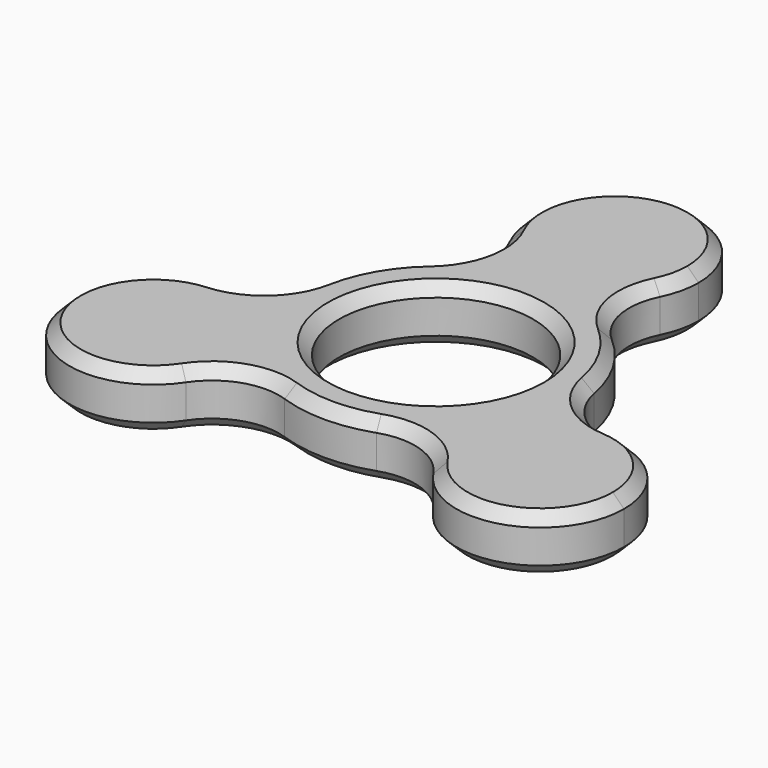
from build123d import *

# Parameters (mm, degrees)
F0_R     = 11.0363
F1_DEPTH = 6.35
F2_SIZE  = 1.27


# Not quite as in the source:
# - a feature names something its author has since deleted; it is built from what else it names


with BuildPart() as f1:
    # F0 (on Top) → F1 (new body)
    with BuildSketch(Plane.XY):
        with BuildLine():
            ThreePointArc((13.7481534459, -7.9374997215), (15.334072534, -4.1087521857), (15.875, 0))
            ThreePointArc((15.875, 0), (15.8042735617, 1.4968507561), (15.592724449, 2.9803639471))
            ThreePointArc((15.592724449, 2.9803639471), (13.7481532851, 7.9375), (10.3774331152, 12.0135135135))
            ThreePointArc((10.3774331152, 12.0135135135), (5.5362937901, 14.8783425176), (-1.09e-08, 15.875))
            ThreePointArc((-1.09e-08, 15.875), (-5.5362938003, 14.8783425138), (-10.3774331152, 12.0135135135))
            ThreePointArc((-10.3774331152, 12.0135135135), (-13.7481532851, 7.9375), (-15.592724449, 2.9803639471))
            ThreePointArc((-15.592724449, 2.9803639471), (-15.6531695071, -2.6446000421), (-13.7481534335, -7.9374997429))
            ThreePointArc((-13.7481534335, -7.9374997429), (-10.1168758016, -12.2337422327), (-5.2152913338, -14.9938774606))
            ThreePointArc((-5.2152913338, -14.9938774606), (0, -15.875), (5.2152913338, -14.9938774606))
            ThreePointArc((5.2152913338, -14.9938774606), (10.1168758111, -12.2337422248), (13.7481534459, -7.9374997215))
        make_face()
        Circle(F0_R, mode=Mode.SUBTRACT)
        with BuildLine():
            ThreePointArc((15.592724449, 2.9803639471), (15.8042735617, 1.4968507561), (15.875, 0))
            ThreePointArc((15.875, 0), (15.334072534, -4.1087521857), (13.7481534459, -7.9374997215))
            ThreePointArc((13.7481534459, -7.9374997215), (17.4968931029, -4.3051053849), (22.5971491052, -3.1939229768))
            ThreePointArc((22.5971491052, -3.1939229768), (18.038469294, -1.3052898819), (15.592724449, 2.9803639471))
        make_face()
        with BuildLine():
            ThreePointArc((14.0645929883, -17.9727436898), (12.4767771707, -13.0002009006), (13.7481534459, -7.9374997215))
            ThreePointArc((13.7481534459, -7.9374997215), (10.1168758111, -12.2337422248), (5.2152913338, -14.9938774606))
            ThreePointArc((5.2152913338, -14.9938774606), (10.149648844, -14.9691277131), (14.0645929883, -17.9727436898))
        make_face()
        with BuildLine():
            ThreePointArc((22.5971491052, -3.1939229768), (17.4968931029, -4.3051053849), (13.7481534459, -7.9374997215))
            ThreePointArc((13.7481534459, -7.9374997215), (12.4767771707, -13.0002009006), (14.0645929883, -17.9727436898))
            ThreePointArc((14.0645929883, -17.9727436898), (24.751043908, -21.81817506), (31.5220452561, -12.7))
            ThreePointArc((31.5220452561, -12.7), (28.9411655806, -6.1804280878), (22.5971491052, -3.1939229768))
        make_face()
        with BuildLine():
            ThreePointArc((-1.09e-08, 15.875), (5.5362937901, 14.8783425176), (10.3774331152, 12.0135135135))
            ThreePointArc((10.3774331152, 12.0135135135), (7.88882045, 16.274417595), (8.5325561169, 21.1666666667))
            ThreePointArc((8.5325561169, 21.1666666667), (5.0201157809, 17.3053065193), (-1.09e-08, 15.875))
        make_face()
        with BuildLine():
            ThreePointArc((-10.3774331152, 12.0135135135), (-5.5362938003, 14.8783425138), (-1.09e-08, 15.875))
            ThreePointArc((-1.09e-08, 15.875), (-5.0201157901, 17.305306525), (-8.5325561169, 21.1666666667))
            ThreePointArc((-8.5325561169, 21.1666666667), (-7.88882045, 16.274417595), (-10.3774331152, 12.0135135135))
        make_face()
        with BuildLine():
            ThreePointArc((-8.5325561169, 21.1666666667), (-5.0201157901, 17.305306525), (-1.09e-08, 15.875))
            ThreePointArc((-1.09e-08, 15.875), (5.0201157809, 17.3053065193), (8.5325561169, 21.1666666667))
            ThreePointArc((8.5325561169, 21.1666666667), (9.2735705641, 23.2259452645), (9.525, 25.4))
            ThreePointArc((9.525, 25.4), (-2.1740547355, 34.6735705641), (-8.5325561169, 21.1666666667))
        make_face()
        with BuildLine():
            ThreePointArc((-14.0645929883, -17.9727436898), (-10.149648844, -14.9691277131), (-5.2152913338, -14.9938774606))
            ThreePointArc((-5.2152913338, -14.9938774606), (-10.1168758016, -12.2337422327), (-13.7481534335, -7.9374997429))
            ThreePointArc((-13.7481534335, -7.9374997429), (-12.7966017991, -10.234748452), (-12.4720452561, -12.7))
            ThreePointArc((-12.4720452561, -12.7), (-12.8788701961, -15.4539986519), (-14.0645929883, -17.9727436898))
        make_face()
        with BuildLine():
            ThreePointArc((-22.5971491052, -3.1939229768), (-17.496893092, -4.3051053908), (-13.7481534335, -7.9374997429))
            ThreePointArc((-13.7481534335, -7.9374997429), (-15.6531695071, -2.6446000421), (-15.592724449, 2.9803639471))
            ThreePointArc((-15.592724449, 2.9803639471), (-18.038469294, -1.3052898819), (-22.5971491052, -3.1939229768))
        make_face()
        with BuildLine():
            ThreePointArc((-12.4720452561, -12.7), (-12.7966017991, -10.234748452), (-13.7481534335, -7.9374997429))
            ThreePointArc((-13.7481534335, -7.9374997429), (-17.496893092, -4.3051053908), (-22.5971491052, -3.1939229768))
            ThreePointArc((-22.5971491052, -3.1939229768), (-30.2459372272, -17.4625), (-14.0645929883, -17.9727436898))
            ThreePointArc((-14.0645929883, -17.9727436898), (-12.8788701961, -15.4539986519), (-12.4720452561, -12.7))
        make_face()
    extrude(amount=F1_DEPTH)

    # F2
    f2_edges = [f1.edges().sort_by_distance(p)[0] for p in [
        (13.748153, 7.9375, 0),
        (7.88882, 16.274418, 0),
        (0, 34.925, 0),
        (-7.88882, 16.274418, 0),
        (-13.748153, 7.9375, 0),
        (-18.038469, -1.30529, 0),
        (-30.245937, -17.4625, 0),
        (-10.149649, -14.969128, 0),
        (0, -15.875, 0),
        (10.149649, -14.969128, 0),
        (30.245937, -17.4625, 0),
        (18.038469, -1.30529, 0),
        (-11.0363, 0, 0),
        (13.748153, 7.9375, 6.35),
        (7.88882, 16.274418, 6.35),
        (0, 34.925, 6.35),
        (-7.88882, 16.274418, 6.35),
        (-13.748153, 7.9375, 6.35),
        (-18.038469, -1.30529, 6.35),
        (-30.245937, -17.4625, 6.35),
        (-10.149649, -14.969128, 6.35),
        (0, -15.875, 6.35),
        (10.149649, -14.969128, 6.35),
        (30.245937, -17.4625, 6.35),
        (18.038469, -1.30529, 6.35),
        (-11.0363, 0, 6.35),
    ]]
    chamfer(f2_edges, length=F2_SIZE)


solid = f1.part
